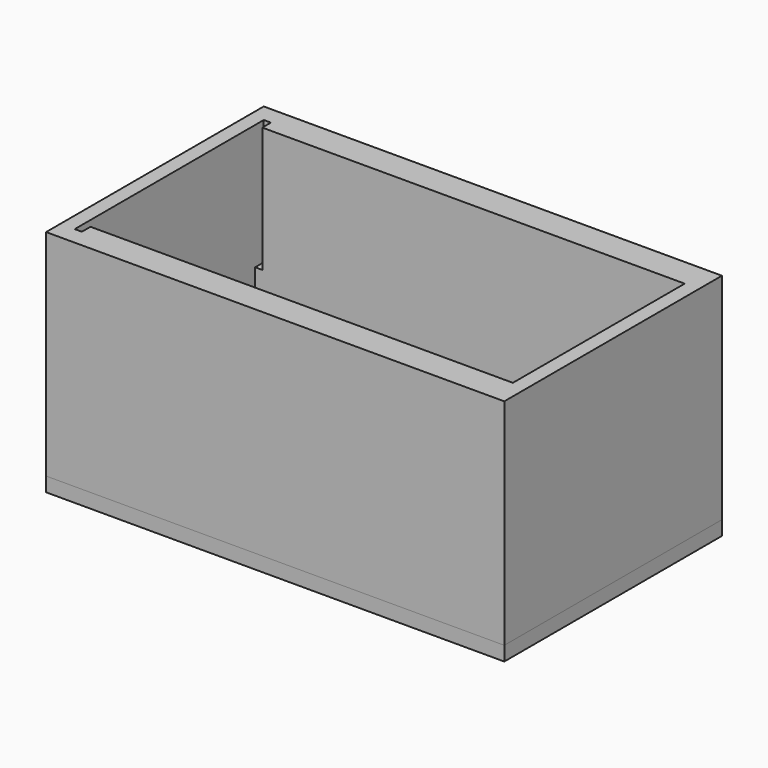
from build123d import *

# Parameters (mm, degrees)
F0_W     = 128
F0_H     = 76
F0_W_2   = 120
F0_H_2   = 60
F1_DEPTH = 60
F2_W     = 2
F2_H     = 3
F3_DEPTH = 35
F4_W     = 128
F4_H     = 76
F5_DEPTH = 4


# Not quite as in the source:
# - a pattern or mirror of a feature is missing from the dataset's text; its kind, count and spacing are read off the source's solid


with BuildPart() as f1:
    # F0 (on Top) → F1 (new body)
    with BuildSketch(Plane.XY):
        Rectangle(F0_W, F0_H)
        Rectangle(F0_W_2, F0_H_2, mode=Mode.SUBTRACT)
    extrude(amount=F1_DEPTH)

    # F2 (on face) → F3 (cut)
    with BuildSketch(Plane.XY.offset(60)):
        with Locations((-59, -31.5)):
            Rectangle(F2_W, F2_H)
    f3 = extrude(amount=-F3_DEPTH, mode=Mode.SUBTRACT)

    # F3_copies: F3 across plane
    add(f3.mirror(Plane.ZX), mode=Mode.SUBTRACT)


with BuildPart() as f5:
    # F4 (on face) → F5 (new body)
    with BuildSketch(Plane(origin=(0, 0, 0), x_dir=(1, 0, 0), z_dir=(0, 0, -1))):
        Rectangle(F4_W, F4_H)
    extrude(amount=F5_DEPTH)


solid = Compound([f1.part, f5.part])
